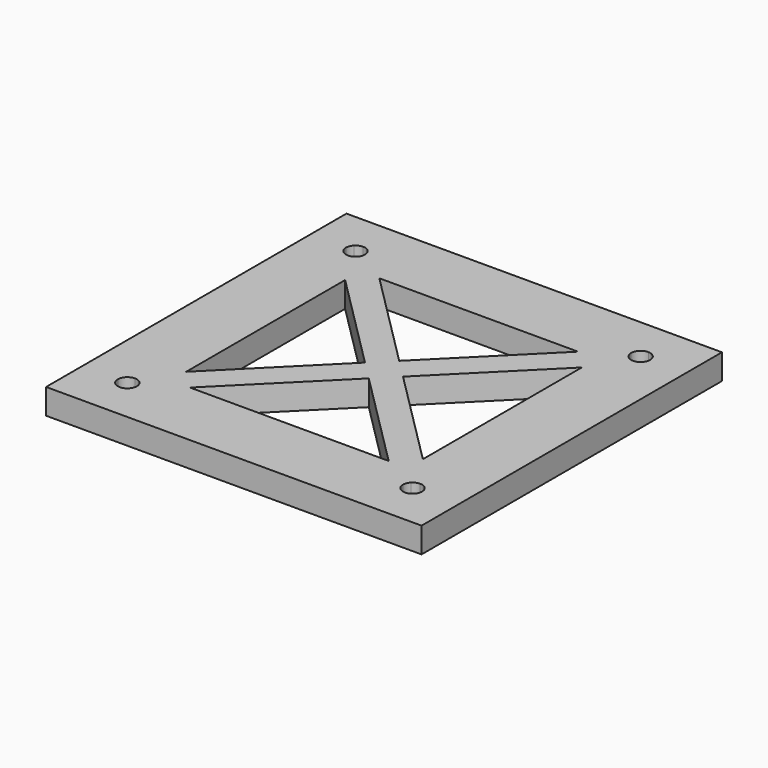
from build123d import *
from build123d import SkipClean  # not in build123d's __all__

# Parameters (mm, degrees)
F0_W     = 3.175
F0_H     = 37.35
F0_W_2   = 37.35
F0_H_2   = 3.175
F1_DEPTH = 4
F2_DEPTH = 2


# Not quite as in the source:
# - a feature names something its author has since deleted; it is built from what else it names


with BuildPart() as f1:
    # F0 (on Top) → F1 (new body)
    with BuildSketch(Plane.XY):
        Polygon((0, -51.35), (-3.95, -55.3), (55.3, -55.3), (51.35, -51.35), (48.175, -51.35), (44.35, -51.35), (7, -51.35), (3.175, -51.35), align=None)
        with Locations((1.5875, -25.675)):
            Rectangle(F0_W, F0_H)
        with Locations((25.675, -49.7625)):
            Rectangle(F0_W_2, F0_H_2)
        with BuildLine():
            Line((3.175, -44.35), (0, -44.35))
            Line((0, -44.35), (0, -48.175))
            Line((0, -48.175), (1.675, -48.175))
            ThreePointArc((1.675, -48.175), (2.1143398282, -47.1143398282), (3.175, -46.675))
            Line((3.175, -46.675), (3.175, -44.35))
        make_face()
        with BuildLine():
            Line((7, -44.35), (3.175, -44.35))
            Line((3.175, -44.35), (3.175, -46.675))
            ThreePointArc((3.175, -46.675), (3.7490251485, -46.7891807012), (4.2356601718, -47.1143398282))
            Line((4.2356601718, -47.1143398282), (7, -44.35))
        make_face()
        with BuildLine():
            Line((2.1143398282, -49.2356601718), (0, -51.35))
            Line((0, -51.35), (3.175, -51.35))
            Line((3.175, -51.35), (3.175, -49.675))
            ThreePointArc((3.175, -49.675), (2.6009748515, -49.5608192988), (2.1143398282, -49.2356601718))
        make_face()
        Polygon((0, -3.175), (0, 0), (-3.95, 3.95), (-3.95, -55.3), (0, -51.35), (0, -48.175), (0, -44.35), (0, -7), align=None)
        Polygon((-3.95, 3.95), (0, 0), (3.175, 0), (7, 0), (44.35, 0), (48.175, 0), (51.35, 0), (55.3, 3.95), align=None)
        with Locations((25.675, -1.5875)):
            Rectangle(F0_W_2, F0_H_2)
        Polygon((55.3, -55.3), (55.3, 3.95), (51.35, 0), (51.35, -3.175), (51.35, -7), (51.35, -44.35), (51.35, -48.175), (51.35, -51.35), align=None)
        with Locations((49.7625, -25.675)):
            Rectangle(F0_W, F0_H)
        with BuildLine():
            Line((49.2356601718, -49.2356601718), (51.35, -51.35))
            Line((51.35, -51.35), (51.35, -48.175))
            Line((51.35, -48.175), (49.675, -48.175))
            ThreePointArc((49.675, -48.175), (49.5608192988, -48.7490251485), (49.2356601718, -49.2356601718))
        make_face()
        with BuildLine():
            Line((49.675, -48.175), (51.35, -48.175))
            Line((51.35, -48.175), (51.35, -44.35))
            Line((51.35, -44.35), (48.175, -44.35))
            Line((48.175, -44.35), (48.175, -46.675))
            ThreePointArc((48.175, -46.675), (49.2356601718, -47.1143398282), (49.675, -48.175))
        make_face()
        with BuildLine():
            Line((48.175, -46.675), (48.175, -44.35))
            Line((48.175, -44.35), (44.35, -44.35))
            Line((44.35, -44.35), (47.1143398282, -47.1143398282))
            ThreePointArc((47.1143398282, -47.1143398282), (47.6009748515, -46.7891807012), (48.175, -46.675))
        make_face()
        Polygon((7, -41.3499998236), (7, -44.35), (8.5000000882, -42.8499999118), align=None)
        Polygon((8.5000000882, -42.8499999118), (7, -44.35), (10.0000001764, -44.35), align=None)
        Polygon((8.5000000882, -42.8499999118), (10.0000001764, -44.35), (25.6750000882, -28.6750000882), (24.175, -27.175), align=None)
        Polygon((22.6749999118, -25.6749999118), (7, -41.3499998236), (8.5000000882, -42.8499999118), (24.175, -27.175), align=None)
        Polygon((8.5, -8.5), (7, -10), (22.6749999118, -25.6749999118), (24.1749999118, -24.1749999118), align=None)
        Polygon((25.6749999118, -22.6749999118), (10, -7), (8.5, -8.5), (24.1749999118, -24.1749999118), align=None)
        Polygon((27.175, -24.175), (25.6749999118, -22.6749999118), (24.1749999118, -24.1749999118), (25.675, -25.675), align=None)
        Polygon((27.1750000882, -27.1750000882), (28.6750000882, -25.6750000882), (27.175, -24.175), (25.675, -25.675), align=None)
        Polygon((25.675, -25.675), (24.175, -27.175), (25.6750000882, -28.6750000882), (27.1750000882, -27.1750000882), align=None)
        Polygon((24.1749999118, -24.1749999118), (22.6749999118, -25.6749999118), (24.175, -27.175), (25.675, -25.675), align=None)
        Polygon((25.6750000882, -28.6750000882), (41.35, -44.35), (42.85, -42.85), (27.1750000882, -27.1750000882), align=None)
        Polygon((42.85, -42.85), (44.35, -41.35), (28.6750000882, -25.6750000882), (27.1750000882, -27.1750000882), align=None)
        Polygon((8.5, -8.5), (7, -7), (7, -10), align=None)
        Polygon((10, -7), (7, -7), (8.5, -8.5), align=None)
        Polygon((28.6750000882, -25.6750000882), (44.35, -10.0000001764), (42.8499999118, -8.5000000882), (27.175, -24.175), align=None)
        Polygon((42.8499999118, -8.5000000882), (41.3499998236, -7), (25.6749999118, -22.6749999118), (27.175, -24.175), align=None)
        Polygon((44.35, -10.0000001764), (44.35, -7), (42.8499999118, -8.5000000882), align=None)
        Polygon((44.35, -44.35), (44.35, -41.35), (42.85, -42.85), align=None)
        Polygon((42.85, -42.85), (41.35, -44.35), (44.35, -44.35), align=None)
        Polygon((42.8499999118, -8.5000000882), (44.35, -7), (41.3499998236, -7), align=None)
        with BuildLine():
            Line((0, -48.175), (0, -51.35))
            Line((0, -51.35), (2.1143398282, -49.2356601718))
            ThreePointArc((2.1143398282, -49.2356601718), (1.7891807012, -48.7490251485), (1.675, -48.175))
            Line((1.675, -48.175), (0, -48.175))
        make_face()
        with BuildLine():
            Line((3.175, -49.675), (3.175, -51.35))
            Line((3.175, -51.35), (7, -51.35))
            Line((7, -51.35), (7, -48.175))
            Line((7, -48.175), (4.675, -48.175))
            ThreePointArc((4.675, -48.175), (4.2356601718, -49.2356601718), (3.175, -49.675))
        make_face()
        with BuildLine():
            Line((7, -48.175), (7, -44.35))
            Line((7, -44.35), (4.2356601718, -47.1143398282))
            ThreePointArc((4.2356601718, -47.1143398282), (4.5608192988, -47.6009748515), (4.675, -48.175))
            Line((4.675, -48.175), (7, -48.175))
        make_face()
        with BuildLine():
            Line((44.35, -51.35), (48.175, -51.35))
            Line((48.175, -51.35), (48.175, -49.675))
            ThreePointArc((48.175, -49.675), (47.1143398282, -49.2356601718), (46.675, -48.175))
            Line((46.675, -48.175), (44.35, -48.175))
            Line((44.35, -48.175), (44.35, -51.35))
        make_face()
        with BuildLine():
            Line((44.35, -44.35), (44.35, -48.175))
            Line((44.35, -48.175), (46.675, -48.175))
            ThreePointArc((46.675, -48.175), (46.7891807012, -47.6009748515), (47.1143398282, -47.1143398282))
            Line((47.1143398282, -47.1143398282), (44.35, -44.35))
        make_face()
        with BuildLine():
            Line((48.175, -51.35), (51.35, -51.35))
            Line((51.35, -51.35), (49.2356601718, -49.2356601718))
            ThreePointArc((49.2356601718, -49.2356601718), (48.7490251485, -49.5608192988), (48.175, -49.675))
            Line((48.175, -49.675), (48.175, -51.35))
        make_face()
        with BuildLine():
            Line((48.175, 0), (44.35, 0))
            Line((44.35, 0), (44.35, -3.175))
            Line((44.35, -3.175), (46.675, -3.175))
            ThreePointArc((46.675, -3.175), (47.1143398282, -2.1143398282), (48.175, -1.675))
            Line((48.175, -1.675), (48.175, 0))
        make_face()
        with BuildLine():
            Line((46.675, -3.175), (44.35, -3.175))
            Line((44.35, -3.175), (44.35, -7))
            Line((44.35, -7), (47.1143398282, -4.2356601718))
            ThreePointArc((47.1143398282, -4.2356601718), (46.7891807012, -3.7490251485), (46.675, -3.175))
        make_face()
        with BuildLine():
            Line((49.2356601718, -2.1143398282), (51.35, 0))
            Line((51.35, 0), (48.175, 0))
            Line((48.175, 0), (48.175, -1.675))
            ThreePointArc((48.175, -1.675), (48.7490251485, -1.7891807012), (49.2356601718, -2.1143398282))
        make_face()
        with BuildLine():
            Line((7, 0), (3.175, 0))
            Line((3.175, 0), (3.175, -1.675))
            ThreePointArc((3.175, -1.675), (4.2356601718, -2.1143398282), (4.675, -3.175))
            Line((4.675, -3.175), (7, -3.175))
            Line((7, -3.175), (7, 0))
        make_face()
        with BuildLine():
            Line((7, -7), (7, -3.175))
            Line((7, -3.175), (4.675, -3.175))
            ThreePointArc((4.675, -3.175), (4.5608192988, -3.7490251485), (4.2356601718, -4.2356601718))
            Line((4.2356601718, -4.2356601718), (7, -7))
        make_face()
        with BuildLine():
            Line((3.175, -4.675), (3.175, -7))
            Line((3.175, -7), (7, -7))
            Line((7, -7), (4.2356601718, -4.2356601718))
            ThreePointArc((4.2356601718, -4.2356601718), (3.7490251485, -4.5608192988), (3.175, -4.675))
        make_face()
        with BuildLine():
            Line((1.675, -3.175), (0, -3.175))
            Line((0, -3.175), (0, -7))
            Line((0, -7), (3.175, -7))
            Line((3.175, -7), (3.175, -4.675))
            ThreePointArc((3.175, -4.675), (2.1143398282, -4.2356601718), (1.675, -3.175))
        make_face()
        with BuildLine():
            Line((2.1143398282, -2.1143398282), (0, 0))
            Line((0, 0), (0, -3.175))
            Line((0, -3.175), (1.675, -3.175))
            ThreePointArc((1.675, -3.175), (1.7891807012, -2.6009748515), (2.1143398282, -2.1143398282))
        make_face()
        Polygon((44.35, -3.175), (7, -3.175), (7, -7), (10, -7), (41.3499998236, -7), (44.35, -7), align=None)
        Polygon((7, -7), (3.175, -7), (3.175, -44.35), (7, -44.35), (7, -41.3499998236), (7, -10), align=None)
        with BuildLine():
            Line((51.35, -3.175), (51.35, 0))
            Line((51.35, 0), (49.2356601718, -2.1143398282))
            ThreePointArc((49.2356601718, -2.1143398282), (49.5608192988, -2.6009748515), (49.675, -3.175))
            Line((49.675, -3.175), (51.35, -3.175))
        make_face()
        with BuildLine():
            Line((51.35, -7), (51.35, -3.175))
            Line((51.35, -3.175), (49.675, -3.175))
            ThreePointArc((49.675, -3.175), (49.2356601718, -4.2356601718), (48.175, -4.675))
            Line((48.175, -4.675), (48.175, -7))
            Line((48.175, -7), (51.35, -7))
        make_face()
        with BuildLine():
            Line((47.1143398282, -4.2356601718), (44.35, -7))
            Line((44.35, -7), (48.175, -7))
            Line((48.175, -7), (48.175, -4.675))
            ThreePointArc((48.175, -4.675), (47.6009748515, -4.5608192988), (47.1143398282, -4.2356601718))
        make_face()
        Polygon((48.175, -7), (44.35, -7), (44.35, -10.0000001764), (44.35, -41.35), (44.35, -44.35), (48.175, -44.35), align=None)
        Polygon((10.0000001764, -44.35), (7, -44.35), (7, -48.175), (44.35, -48.175), (44.35, -44.35), (41.35, -44.35), align=None)
        with BuildLine():
            Line((3.175, 0), (0, 0))
            Line((0, 0), (2.1143398282, -2.1143398282))
            ThreePointArc((2.1143398282, -2.1143398282), (2.6009748515, -1.7891807012), (3.175, -1.675))
            Line((3.175, -1.675), (3.175, 0))
        make_face()
    extrude(amount=F1_DEPTH)

    # F0 (on Top) → F2 (join)
    with BuildSketch(Plane.XY):
        with BuildLine():
            Line((3.175, -44.35), (0, -44.35))
            Line((0, -44.35), (0, -48.175))
            Line((0, -48.175), (1.675, -48.175))
            ThreePointArc((1.675, -48.175), (2.1143398282, -47.1143398282), (3.175, -46.675))
            Line((3.175, -46.675), (3.175, -44.35))
        make_face()
        with BuildLine():
            Line((7, -44.35), (3.175, -44.35))
            Line((3.175, -44.35), (3.175, -46.675))
            ThreePointArc((3.175, -46.675), (3.7490251485, -46.7891807012), (4.2356601718, -47.1143398282))
            Line((4.2356601718, -47.1143398282), (7, -44.35))
        make_face()
        with BuildLine():
            Line((2.1143398282, -49.2356601718), (0, -51.35))
            Line((0, -51.35), (3.175, -51.35))
            Line((3.175, -51.35), (3.175, -49.675))
            ThreePointArc((3.175, -49.675), (2.6009748515, -49.5608192988), (2.1143398282, -49.2356601718))
        make_face()
        with BuildLine():
            Line((49.675, -48.175), (51.35, -48.175))
            Line((51.35, -48.175), (51.35, -44.35))
            Line((51.35, -44.35), (48.175, -44.35))
            Line((48.175, -44.35), (48.175, -46.675))
            ThreePointArc((48.175, -46.675), (49.2356601718, -47.1143398282), (49.675, -48.175))
        make_face()
        with BuildLine():
            Line((48.175, -46.675), (48.175, -44.35))
            Line((48.175, -44.35), (44.35, -44.35))
            Line((44.35, -44.35), (47.1143398282, -47.1143398282))
            ThreePointArc((47.1143398282, -47.1143398282), (47.6009748515, -46.7891807012), (48.175, -46.675))
        make_face()
        with BuildLine():
            Line((49.2356601718, -49.2356601718), (51.35, -51.35))
            Line((51.35, -51.35), (51.35, -48.175))
            Line((51.35, -48.175), (49.675, -48.175))
            ThreePointArc((49.675, -48.175), (49.5608192988, -48.7490251485), (49.2356601718, -49.2356601718))
        make_face()
        with BuildLine():
            Line((3.175, -49.675), (3.175, -51.35))
            Line((3.175, -51.35), (7, -51.35))
            Line((7, -51.35), (7, -48.175))
            Line((7, -48.175), (4.675, -48.175))
            ThreePointArc((4.675, -48.175), (4.2356601718, -49.2356601718), (3.175, -49.675))
        make_face()
        with BuildLine():
            Line((7, -48.175), (7, -44.35))
            Line((7, -44.35), (4.2356601718, -47.1143398282))
            ThreePointArc((4.2356601718, -47.1143398282), (4.5608192988, -47.6009748515), (4.675, -48.175))
            Line((4.675, -48.175), (7, -48.175))
        make_face()
        with BuildLine():
            Line((0, -48.175), (0, -51.35))
            Line((0, -51.35), (2.1143398282, -49.2356601718))
            ThreePointArc((2.1143398282, -49.2356601718), (1.7891807012, -48.7490251485), (1.675, -48.175))
            Line((1.675, -48.175), (0, -48.175))
        make_face()
        with BuildLine():
            Line((44.35, -51.35), (48.175, -51.35))
            Line((48.175, -51.35), (48.175, -49.675))
            ThreePointArc((48.175, -49.675), (47.1143398282, -49.2356601718), (46.675, -48.175))
            Line((46.675, -48.175), (44.35, -48.175))
            Line((44.35, -48.175), (44.35, -51.35))
        make_face()
        with BuildLine():
            Line((44.35, -44.35), (44.35, -48.175))
            Line((44.35, -48.175), (46.675, -48.175))
            ThreePointArc((46.675, -48.175), (46.7891807012, -47.6009748515), (47.1143398282, -47.1143398282))
            Line((47.1143398282, -47.1143398282), (44.35, -44.35))
        make_face()
        with BuildLine():
            Line((48.175, -51.35), (51.35, -51.35))
            Line((51.35, -51.35), (49.2356601718, -49.2356601718))
            ThreePointArc((49.2356601718, -49.2356601718), (48.7490251485, -49.5608192988), (48.175, -49.675))
            Line((48.175, -49.675), (48.175, -51.35))
        make_face()
        with BuildLine():
            Line((48.175, 0), (44.35, 0))
            Line((44.35, 0), (44.35, -3.175))
            Line((44.35, -3.175), (46.675, -3.175))
            ThreePointArc((46.675, -3.175), (47.1143398282, -2.1143398282), (48.175, -1.675))
            Line((48.175, -1.675), (48.175, 0))
        make_face()
        with BuildLine():
            Line((46.675, -3.175), (44.35, -3.175))
            Line((44.35, -3.175), (44.35, -7))
            Line((44.35, -7), (47.1143398282, -4.2356601718))
            ThreePointArc((47.1143398282, -4.2356601718), (46.7891807012, -3.7490251485), (46.675, -3.175))
        make_face()
        with BuildLine():
            Line((49.2356601718, -2.1143398282), (51.35, 0))
            Line((51.35, 0), (48.175, 0))
            Line((48.175, 0), (48.175, -1.675))
            ThreePointArc((48.175, -1.675), (48.7490251485, -1.7891807012), (49.2356601718, -2.1143398282))
        make_face()
        with BuildLine():
            Line((1.675, -3.175), (0, -3.175))
            Line((0, -3.175), (0, -7))
            Line((0, -7), (3.175, -7))
            Line((3.175, -7), (3.175, -4.675))
            ThreePointArc((3.175, -4.675), (2.1143398282, -4.2356601718), (1.675, -3.175))
        make_face()
        with BuildLine():
            Line((3.175, -4.675), (3.175, -7))
            Line((3.175, -7), (7, -7))
            Line((7, -7), (4.2356601718, -4.2356601718))
            ThreePointArc((4.2356601718, -4.2356601718), (3.7490251485, -4.5608192988), (3.175, -4.675))
        make_face()
        with BuildLine():
            Line((7, -7), (7, -3.175))
            Line((7, -3.175), (4.675, -3.175))
            ThreePointArc((4.675, -3.175), (4.5608192988, -3.7490251485), (4.2356601718, -4.2356601718))
            Line((4.2356601718, -4.2356601718), (7, -7))
        make_face()
        with BuildLine():
            Line((3.175, 0), (0, 0))
            Line((0, 0), (2.1143398282, -2.1143398282))
            ThreePointArc((2.1143398282, -2.1143398282), (2.6009748515, -1.7891807012), (3.175, -1.675))
            Line((3.175, -1.675), (3.175, 0))
        make_face()
        with BuildLine():
            Line((2.1143398282, -2.1143398282), (0, 0))
            Line((0, 0), (0, -3.175))
            Line((0, -3.175), (1.675, -3.175))
            ThreePointArc((1.675, -3.175), (1.7891807012, -2.6009748515), (2.1143398282, -2.1143398282))
        make_face()
        with BuildLine():
            Line((7, 0), (3.175, 0))
            Line((3.175, 0), (3.175, -1.675))
            ThreePointArc((3.175, -1.675), (4.2356601718, -2.1143398282), (4.675, -3.175))
            Line((4.675, -3.175), (7, -3.175))
            Line((7, -3.175), (7, 0))
        make_face()
        with BuildLine():
            Line((51.35, -3.175), (51.35, 0))
            Line((51.35, 0), (49.2356601718, -2.1143398282))
            ThreePointArc((49.2356601718, -2.1143398282), (49.5608192988, -2.6009748515), (49.675, -3.175))
            Line((49.675, -3.175), (51.35, -3.175))
        make_face()
        with BuildLine():
            Line((51.35, -7), (51.35, -3.175))
            Line((51.35, -3.175), (49.675, -3.175))
            ThreePointArc((49.675, -3.175), (49.2356601718, -4.2356601718), (48.175, -4.675))
            Line((48.175, -4.675), (48.175, -7))
            Line((48.175, -7), (51.35, -7))
        make_face()
        with BuildLine():
            Line((47.1143398282, -4.2356601718), (44.35, -7))
            Line((44.35, -7), (48.175, -7))
            Line((48.175, -7), (48.175, -4.675))
            ThreePointArc((48.175, -4.675), (47.6009748515, -4.5608192988), (47.1143398282, -4.2356601718))
        make_face()
    with SkipClean():  # cleaning this boolean's faces spoils the solid; the shape is the same uncleaned
        extrude(amount=-F2_DEPTH)


solid = f1.part
